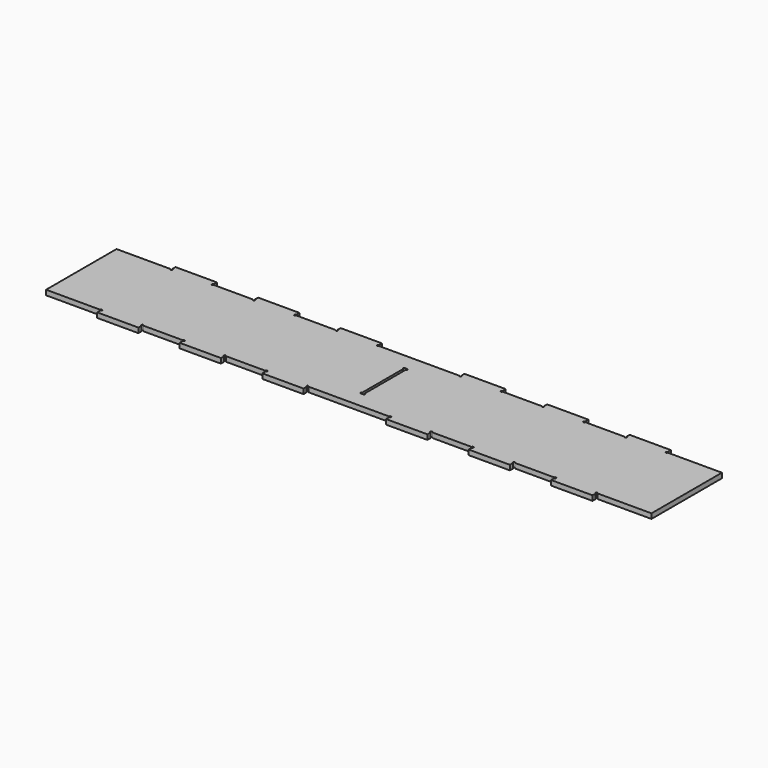
from build123d import *

# Parameters (mm, degrees)
F1_DEPTH = 18
F2_DEPTH = 9


# Not quite as in the source:
# - ends of sketch curves that miss each other by under 0.0002 mm in the source are joined


with BuildPart() as f1:
    # F0 (on Top) → F1 (new body)
    with BuildSketch(Plane.XY):
        with BuildLine():
            Line((-1127.3931139915, 97.8692322969), (-1127.3931139915, -62.1307669387))
            Line((-1127.3931139915, -62.1307669387), (-930.8931139915, -62.1307669387))
            ThreePointArc((-930.8931139915, -62.1307669387), (-924.9182402574, -59.6558932046), (-927.3931139915, -65.6307669387))
            Line((-927.3931139915, -65.6307669387), (-927.3931139915, -80.1307669387))
            Line((-927.3931139915, -80.1307669387), (-777.3931378334, -80.1307669387))
            Line((-777.3931378334, -80.1307669387), (-777.3931378334, -65.6307669387))
            ThreePointArc((-777.3931378334, -65.6307669387), (-779.8680115675, -59.6558932046), (-773.8931378334, -62.1307669387))
            Line((-773.8931378334, -62.1307669387), (-630.8931139915, -62.1307669387))
            ThreePointArc((-630.8931139915, -62.1307669387), (-624.9182402574, -59.6558932046), (-627.3931139915, -65.6307669387))
            Line((-627.3931139915, -65.6307669387), (-627.3931139915, -80.1307669387))
            Line((-627.3931139915, -80.1307669387), (-477.3931378334, -80.1307669387))
            Line((-477.3931378334, -80.1307669387), (-477.3931378334, -65.6307669387))
            ThreePointArc((-477.3931378334, -65.6307669387), (-479.8680115675, -59.6558932046), (-473.8931378334, -62.1307669387))
            Line((-473.8931378334, -62.1307669387), (-330.8931139915, -62.1307669387))
            ThreePointArc((-330.8931139915, -62.1307669387), (-324.9182402574, -59.6558932046), (-327.3931139915, -65.6307669387))
            Line((-327.3931139915, -65.6307669387), (-327.3931139915, -80.1307669387))
            Line((-327.3931139915, -80.1307669387), (-177.3931378334, -80.1307669387))
            Line((-177.3931378334, -80.1307669387), (-177.3931378334, -65.6307669387))
            ThreePointArc((-177.3931378334, -65.6307669387), (-179.8680115675, -59.6558932046), (-173.8931378334, -62.1307669387))
            Line((-173.8931378334, -62.1307669387), (-27.3931378334, -62.1307669387))
            Line((-27.3931378334, -62.1307669387), (119.1069098503, -62.1307669387))
            ThreePointArc((119.1069098503, -62.1307669387), (125.0817835845, -59.6558932046), (122.6069098503, -65.6307669387))
            Line((122.6069098503, -65.6307669387), (122.6069098503, -80.1307669387))
            Line((122.6069098503, -80.1307669387), (272.6068860085, -80.1307669387))
            Line((272.6068860085, -80.1307669387), (272.6068860085, -65.6307669387))
            ThreePointArc((272.6068860085, -65.6307669387), (270.1320122743, -59.6558932046), (276.1068860085, -62.1307669387))
            Line((276.1068860085, -62.1307669387), (419.1069098503, -62.1307669387))
            ThreePointArc((419.1069098503, -62.1307669387), (425.0817835845, -59.6558932046), (422.6069098503, -65.6307669387))
            Line((422.6069098503, -65.6307669387), (422.6069098503, -80.1307669387))
            Line((422.6069098503, -80.1307669387), (572.6068860085, -80.1307669387))
            Line((572.6068860085, -80.1307669387), (572.6068860085, -65.6307669387))
            ThreePointArc((572.6068860085, -65.6307669387), (570.1320122743, -59.6558932046), (576.1068860085, -62.1307669387))
            Line((576.1068860085, -62.1307669387), (719.1069098503, -62.1307669387))
            ThreePointArc((719.1069098503, -62.1307669387), (725.0817835845, -59.6558932046), (722.6069098503, -65.6307669387))
            Line((722.6069098503, -65.6307669387), (722.6069098503, -80.1307669387))
            Line((722.6069098503, -80.1307669387), (872.6068860085, -80.1307669387))
            Line((872.6068860085, -80.1307669387), (872.6068860085, -65.6307669387))
            ThreePointArc((872.6068860085, -65.6307669387), (870.1320122743, -59.6558932046), (876.1068860085, -62.1307669387))
            Line((876.1068860085, -62.1307669387), (1072.6068860085, -62.1307669387))
            Line((1072.6068860085, -62.1307669387), (1072.6068860085, 97.8692322969))
            Line((1072.6068860085, 97.8692322969), (1072.6068860085, 257.8692315326))
            Line((1072.6068860085, 257.8692315326), (876.1068860085, 257.8692315326))
            ThreePointArc((876.1068860085, 257.8692315326), (870.1320122743, 255.3943577985), (872.6068860085, 261.3692315326))
            Line((872.6068860085, 261.3692315326), (872.6068860085, 275.8692315326))
            Line((872.6068860085, 275.8692315326), (722.6069098503, 275.8692315326))
            Line((722.6069098503, 275.8692315326), (722.6069098503, 261.3692315326))
            ThreePointArc((722.6069098503, 261.3692315326), (725.0817835845, 255.3943577985), (719.1069098503, 257.8692315326))
            Line((719.1069098503, 257.8692315326), (576.1068860085, 257.8692315326))
            ThreePointArc((576.1068860085, 257.8692315326), (570.1320122743, 255.3943577985), (572.6068860085, 261.3692315326))
            Line((572.6068860085, 261.3692315326), (572.6068860085, 275.8692315326))
            Line((572.6068860085, 275.8692315326), (422.6069098503, 275.8692315326))
            Line((422.6069098503, 275.8692315326), (422.6069098503, 261.3692315326))
            ThreePointArc((422.6069098503, 261.3692315326), (425.0817835845, 255.3943577985), (419.1069098503, 257.8692315326))
            Line((419.1069098503, 257.8692315326), (276.1068860085, 257.8692315326))
            ThreePointArc((276.1068860085, 257.8692315326), (270.1320122743, 255.3943577985), (272.6068860085, 261.3692315326))
            Line((272.6068860085, 261.3692315326), (272.6068860085, 275.8692315326))
            Line((272.6068860085, 275.8692315326), (122.6069098503, 275.8692315326))
            Line((122.6069098503, 275.8692315326), (122.6069098503, 261.3692315326))
            ThreePointArc((122.6069098503, 261.3692315326), (125.0817835845, 255.3943577985), (119.1069098503, 257.8692315326))
            Line((119.1069098503, 257.8692315326), (-27.3930901497, 257.8692315326))
            Line((-27.3930901497, 257.8692315326), (-173.8931378334, 257.8692315326))
            ThreePointArc((-173.8931378334, 257.8692315326), (-179.8680115675, 255.3943577985), (-177.3931378334, 261.3692315326))
            Line((-177.3931378334, 261.3692315326), (-177.3931378334, 275.8692315326))
            Line((-177.3931378334, 275.8692315326), (-327.3931139915, 275.8692315326))
            Line((-327.3931139915, 275.8692315326), (-327.3931139915, 261.3692315326))
            ThreePointArc((-327.3931139915, 261.3692315326), (-324.9182402574, 255.3943577985), (-330.8931139915, 257.8692315326))
            Line((-330.8931139915, 257.8692315326), (-473.8931378334, 257.8692315326))
            ThreePointArc((-473.8931378334, 257.8692315326), (-479.8680115675, 255.3943577985), (-477.3931378334, 261.3692315326))
            Line((-477.3931378334, 261.3692315326), (-477.3931378334, 275.8692315326))
            Line((-477.3931378334, 275.8692315326), (-627.3931139915, 275.8692315326))
            Line((-627.3931139915, 275.8692315326), (-627.3931139915, 261.3692315326))
            ThreePointArc((-627.3931139915, 261.3692315326), (-624.9182402574, 255.3943577985), (-630.8931139915, 257.8692315326))
            Line((-630.8931139915, 257.8692315326), (-773.8931378334, 257.8692315326))
            ThreePointArc((-773.8931378334, 257.8692315326), (-779.8680115675, 255.3943577985), (-777.3931378334, 261.3692315326))
            Line((-777.3931378334, 261.3692315326), (-777.3931378334, 275.8692315326))
            Line((-777.3931378334, 275.8692315326), (-927.3931139915, 275.8692315326))
            Line((-927.3931139915, 275.8692315326), (-927.3931139915, 261.3692315326))
            ThreePointArc((-927.3931139915, 261.3692315326), (-924.9182402574, 255.3943577985), (-930.8931139915, 257.8692315326))
            Line((-930.8931139915, 257.8692315326), (-1127.3931139915, 257.8692315326))
            Line((-1127.3931139915, 257.8692315326), (-1127.3931139915, 97.8692322969))
        make_face()
        with BuildLine():
            Line((-22.8931139915, 190.8692322969), (-22.8931139915, 97.8692322969))
            Line((-22.8931139915, 97.8692322969), (-22.8931139915, 4.8692322969))
            ThreePointArc((-22.8931139915, 4.8692322969), (-19.3931139915, 1.3692322969), (-22.8931139915, -2.1307677031))
            Line((-22.8931139915, -2.1307677031), (-27.3931139915, -2.1307677031))
            Line((-27.3931139915, -2.1307677031), (-31.8931139915, -2.1307677031))
            ThreePointArc((-31.8931139915, -2.1307677031), (-35.3931139915, 1.3692322969), (-31.8931139915, 4.8692322969))
            Line((-31.8931139915, 4.8692322969), (-31.8931139915, 97.8692322969))
            Line((-31.8931139915, 97.8692322969), (-31.8931139915, 190.8692322969))
            ThreePointArc((-31.8931139915, 190.8692322969), (-35.3931139915, 194.3692322969), (-31.8931139915, 197.8692322969))
            Line((-31.8931139915, 197.8692322969), (-27.3931139915, 197.8692322969))
            Line((-27.3931139915, 197.8692322969), (-22.8931139915, 197.8692322969))
            ThreePointArc((-22.8931139915, 197.8692322969), (-19.3931139915, 194.3692322969), (-22.8931139915, 190.8692322969))
        make_face(mode=Mode.SUBTRACT)
    extrude(amount=F1_DEPTH)

    # F0 (on Top) → F2 (join)
    with BuildSketch(Plane.XY):
        with BuildLine():
            Line((-22.8931139915, 4.8692322969), (-22.8931139915, 97.8692322969))
            Line((-22.8931139915, 97.8692322969), (-22.8931139915, 190.8692322969))
            ThreePointArc((-22.8931139915, 190.8692322969), (-19.3931139915, 194.3692322969), (-22.8931139915, 197.8692322969))
            Line((-22.8931139915, 197.8692322969), (-27.3931139915, 197.8692322969))
            Line((-27.3931139915, 197.8692322969), (-31.8931139915, 197.8692322969))
            ThreePointArc((-31.8931139915, 197.8692322969), (-35.3931139915, 194.3692322969), (-31.8931139915, 190.8692322969))
            Line((-31.8931139915, 190.8692322969), (-31.8931139915, 97.8692322969))
            Line((-31.8931139915, 97.8692322969), (-31.8931139915, 4.8692322969))
            ThreePointArc((-31.8931139915, 4.8692322969), (-35.3931139915, 1.3692322969), (-31.8931139915, -2.1307677031))
            Line((-31.8931139915, -2.1307677031), (-27.3931139915, -2.1307677031))
            Line((-27.3931139915, -2.1307677031), (-22.8931139915, -2.1307677031))
            ThreePointArc((-22.8931139915, -2.1307677031), (-19.3931139915, 1.3692322969), (-22.8931139915, 4.8692322969))
        make_face()
    extrude(amount=F2_DEPTH)


solid = f1.part
